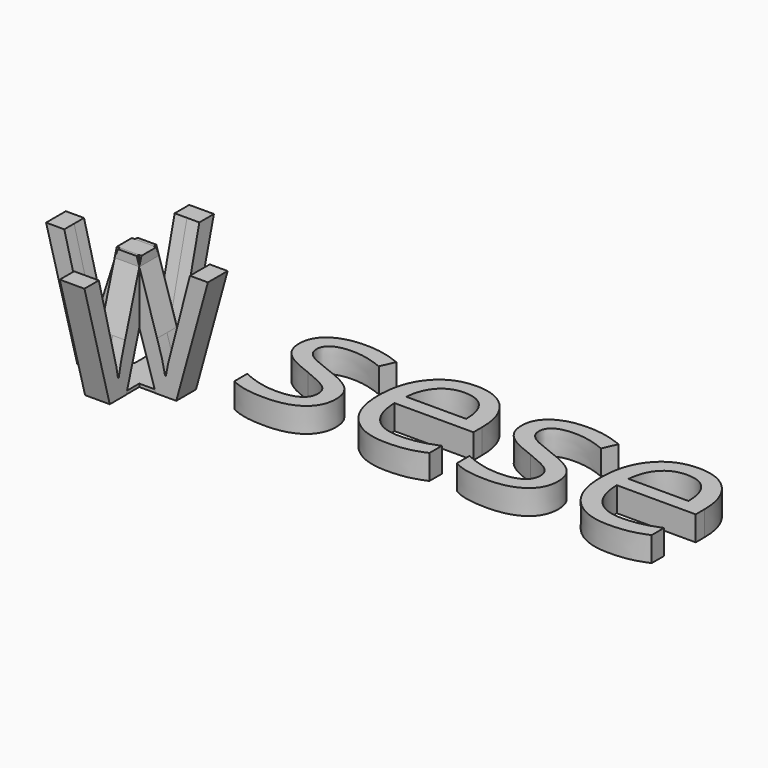
from build123d import *

# Parameters (mm, degrees)
F0_TEXT_SIZE  = 34.7222222222
F1_DEPTH      = 2
F1_DEPTH_BACK = 2
F3_COUNT      = 2
F3_ANGLE      = 90
F4_TEXT_SIZE  = 34.7222222222
F5_DEPTH      = 4
F7_DEPTH      = 0.5


# Not quite as in the source:
# - Text() gives the source's letters only with a copy of the font that has no kerning and outlines rounded to 1/6400 em; it was checked with that copy


with BuildPart() as f1:
    # F0 (on Front) → F1 (new body, two sides)
    with BuildSketch(Plane.XZ) as f1_sk:
        with Locations((-13.5088135971, 0)):
            Text('w', F0_TEXT_SIZE, font='Open Sans', text_align=(TextAlign.LEFT, TextAlign.BOTTOM))
    extrude(amount=F1_DEPTH)
    extrude(f1_sk.sketch, amount=-F1_DEPTH_BACK)


with BuildPart() as f3_1:
    # F3: instance of F1
    add(f1.part.rotate(Axis((0, 0, 2.2740624845), (0, 0, -1)), 1 * F3_ANGLE / (F3_COUNT - 1)))


with BuildPart() as f5:
    # F4 (on Top) → F5 (new body)
    with BuildSketch(Plane.XY):
        with Locations((13.319967993, 0)):
            Text('sese', F4_TEXT_SIZE, font='Open Sans', text_align=(TextAlign.LEFT, TextAlign.BOTTOM))
    extrude(amount=F5_DEPTH)


with BuildPart() as f7:
    # F6 (on face) → F7 (new body)
    with BuildSketch(Plane(origin=(0, 0, 0), x_dir=(1, 0, 0), z_dir=(0, 0, -1))):
        Polygon((-1.996894367, 1.9701521452), (-8.0499053001, 1.9701521452), (-8.0499053001, -1.996894367), (-1.996894367, -1.996894367), (-1.996894367, -7.9744842369), (1.9701521452, -7.9744842369), (1.9701521452, -1.996894367), (7.9744842369, -1.996894367), (7.9744842369, 1.9701521452), (1.9701521452, 1.9701521452), (1.9701521452, 4.6498235557), (-1.996894367, 4.6498235557), align=None)
    extrude(amount=-F7_DEPTH)


solid = Compound([f1.part, f3_1.part, f5.part, f7.part])
